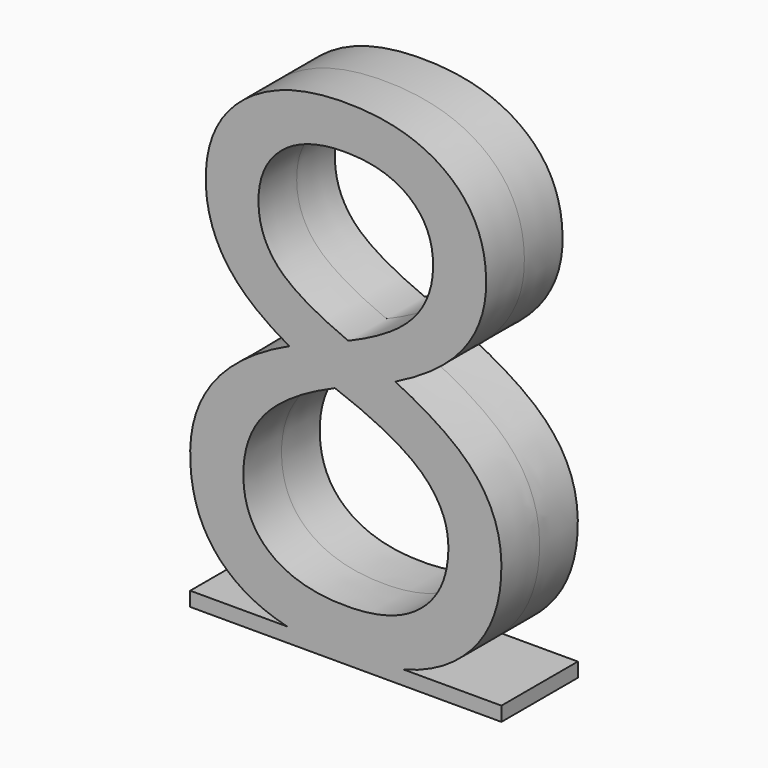
from build123d import *

# Parameters (mm, degrees)
F0_TEXT_SIZE  = 138.8888888889
F1_DEPTH      = 10
F1_DEPTH_BACK = 10
F2_W          = 65.1692708333
F2_H          = 20
F3_DEPTH      = 3


# Not quite as in the source:
# - Text() gives the source's letters only with a copy of the font that has no kerning and outlines rounded to 1/6400 em; it was checked with that copy


with BuildPart() as f1:
    # F0 (on Front) → F1 (new body, two sides)
    with BuildSketch(Plane.XZ) as f1_sk:
        with Locations((-40.6141493056, 0)):
            Text('8', F0_TEXT_SIZE, font='Open Sans', text_align=(TextAlign.LEFT, TextAlign.BOTTOM))
    extrude(amount=F1_DEPTH)
    extrude(f1_sk.sketch, amount=-F1_DEPTH_BACK)

    # F2 (on Top) → F3 (join)
    with BuildSketch(Plane.XY):
        with Locations((-0.9765625, 0)):
            Rectangle(F2_W, F2_H)
    extrude(amount=-F3_DEPTH)


solid = f1.part
